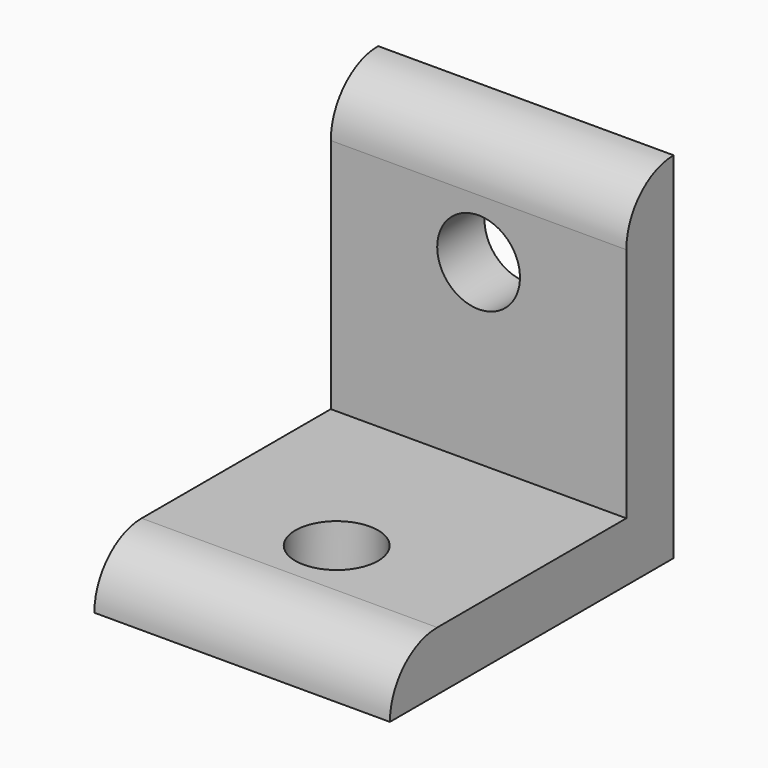
from build123d import *

# Parameters (mm, degrees)
F0_W     = 25
F0_H     = 25
F0_R     = 3.5
F1_DEPTH = 5
F0_H_2   = 5
F2_DEPTH = 30
F3_R     = 3.5
F4_DEPTH = 5
F5_R     = 4.99999
F6_R     = 4.99999


# Not quite as in the source:
# - a fillet or chamfer is up to 0.001 mm smaller than in the source, because OpenCascade refuses the exact size


with BuildPart() as f1:
    # F0 (on Top) → F1 (new body)
    with BuildSketch(Plane.XY):
        with Locations((0, -2.5)):
            Rectangle(F0_W, F0_H)
        with Locations((0, -5)):
            Circle(F0_R, mode=Mode.SUBTRACT)
    extrude(amount=F1_DEPTH)

    # F0 (on Top) → F2 (join)
    with BuildSketch(Plane.XY):
        with Locations((0, 12.5)):
            Rectangle(F0_W, F0_H_2)
    extrude(amount=F2_DEPTH)

    # F3 (on face) → F4 (cut)
    with BuildSketch(Plane(origin=(0, 15, 0), x_dir=(-1, 0, 0), z_dir=(0, 1, 0))):
        with Locations((0, 20)):
            Circle(F3_R)
    extrude(amount=-F4_DEPTH, mode=Mode.SUBTRACT)

    # F5 (radius 5 in the source; OpenCascade refuses exactly that, so slightly less here)
    f5_edges = [f1.edges().sort_by_distance(p)[0] for p in [
        (0, 10, 30),
    ]]
    fillet(f5_edges, radius=F5_R)

    # F6 (radius 5 in the source; OpenCascade refuses exactly that, so slightly less here)
    f6_edges = [f1.edges().sort_by_distance(p)[0] for p in [
        (0, -15, 5),
    ]]
    fillet(f6_edges, radius=F6_R)


solid = f1.part
